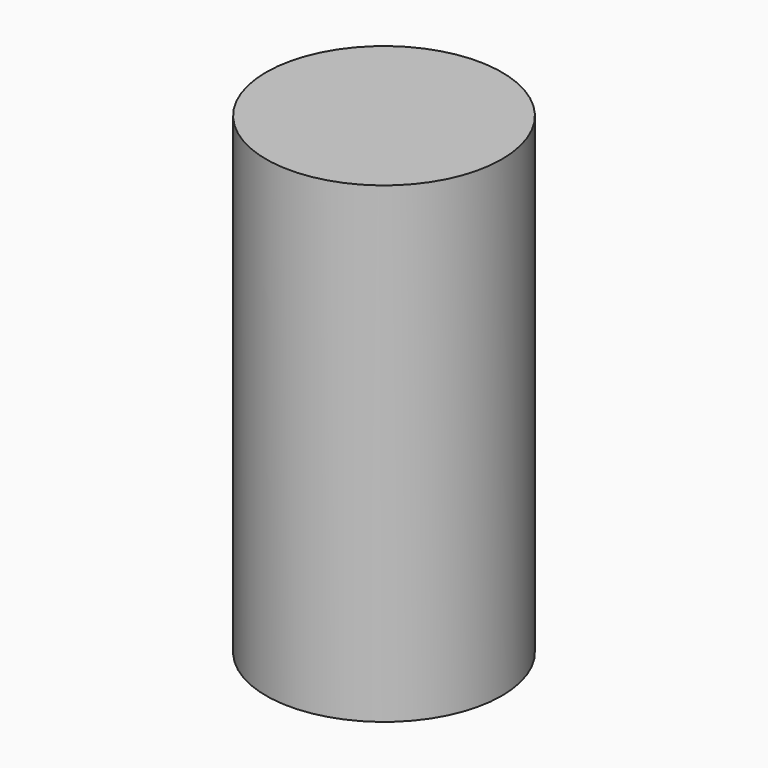
from build123d import *

# Parameters (mm, degrees)
F0_R     = 11.2
F0_R_2   = 2.02
F2_DEPTH = 44.88


# Not quite as in the source:
# - the program builds the solid bodies; features that only make, move or delete a surface that nothing else refers to are left out


with BuildPart() as f2:
    # F0 (on Top) → F2 (new body)
    with BuildSketch(Plane.XY):
        Circle(F0_R)
        Circle(F0_R_2, mode=Mode.SUBTRACT)
        Circle(F0_R_2)
    extrude(amount=F2_DEPTH)


solid = f2.part
